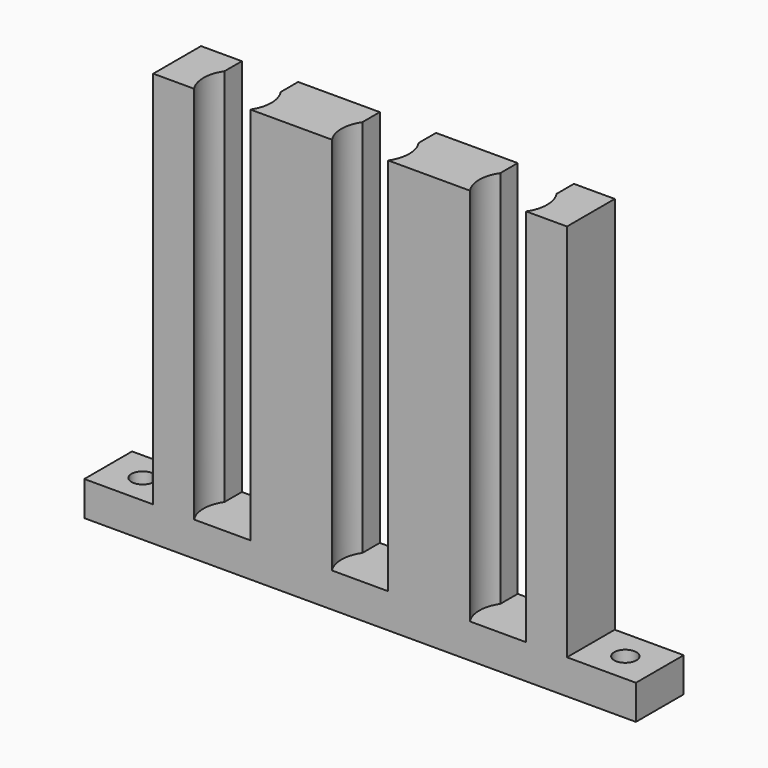
from build123d import *

# Parameters (mm, degrees)
F0_W         = 76.2
F0_H         = 11
F1_DEPTH     = 76.2
F2_R         = 6.25
F3_DEPTH     = 69.85
F4_TEXT_SIZE = 5.2916666667
F5_DEPTH     = 0.5
F6_W         = 11
F6_H         = 6.35
F7_DEPTH     = 12.7
F8_W         = 11
F8_H         = 6.35
F9_DEPTH     = 12.7
F10_R        = 2.05
F11_DEPTH    = 6.35
F12_W        = 10.3561575886
F12_H        = 4
F13_DEPTH    = 69.85


# Not quite as in the source:
# - Text() gives the source's letters only with a copy of the font that has no kerning and outlines rounded to 1/6400 em; it was checked with that copy


with BuildPart() as f1:
    # F0 (on Top) → F1 (new body)
    with BuildSketch(Plane.XY):
        Rectangle(F0_W, F0_H)
    extrude(amount=F1_DEPTH)

    # F2 (on face) → F3 (cut)
    with BuildSketch(Plane.XY.offset(76.2)):
        with BuildLine():
            ThreePointArc((0, 4.25), (-4.4194173824, -6.4194173824), (6.25, -2))
            ThreePointArc((6.25, -2), (4.4194173824, 2.4194173824), (0, 4.25))
        make_face()
        with Locations((-25.4, -2)):
            Circle(F2_R)
        with Locations((25.4, -2)):
            Circle(F2_R)
    extrude(amount=-F3_DEPTH, mode=Mode.SUBTRACT)

    # F4 (on face) → F5 (cut)
    with BuildSketch(Plane(origin=(0, 5.5, 0), x_dir=(-1, 0, 0), z_dir=(0, 1, 0))):
        with Locations((-26.8469244572, 1.5566079867)):
            Text('1', F4_TEXT_SIZE, font='Open Sans', text_align=(TextAlign.LEFT, TextAlign.BOTTOM))
        with Locations((-1.5416732874, 1.5566079867)):
            Text('2', F4_TEXT_SIZE, font='Open Sans', text_align=(TextAlign.LEFT, TextAlign.BOTTOM))
        with Locations((24.0893187388, 1.5566079867)):
            Text('3', F4_TEXT_SIZE, font='Open Sans', text_align=(TextAlign.LEFT, TextAlign.BOTTOM))
    extrude(amount=-F5_DEPTH, mode=Mode.SUBTRACT)

    # F6 (on face) → F7 (join)
    with BuildSketch(Plane.YZ.offset(38.1)):
        with Locations((0, 3.175)):
            Rectangle(F6_W, F6_H)
    extrude(amount=F7_DEPTH)

    # F8 (on face) → F9 (join)
    with BuildSketch(Plane(origin=(-38.1, 0, 0), x_dir=(0, -1, 0), z_dir=(-1, 0, 0))):
        with Locations((0, 3.175)):
            Rectangle(F8_W, F8_H)
    extrude(amount=F9_DEPTH)

    # F10 (on face) → F11 (cut, through all)
    with BuildSketch(Plane.XY.offset(6.35)):
        with BuildLine():
            ThreePointArc((-44.45, -2.05), (-43.0004310986, -1.4495689014), (-42.4, 0))
            ThreePointArc((-42.4, 0), (-43.0004310986, 1.4495689014), (-44.45, 2.05))
            Line((-44.45, 2.05), (-44.45, -2.05))
        make_face()
        with BuildLine():
            Line((-44.45, -2.05), (-44.45, 2.05))
            ThreePointArc((-44.45, 2.05), (-46.5, 0), (-44.45, -2.05))
        make_face()
        with Locations((44.45, 0)):
            Circle(F10_R)
    extrude(amount=-F11_DEPTH, mode=Mode.SUBTRACT)

    # F12 (on face) → F13 (cut, through all)
    with BuildSketch(Plane.XY.offset(76.2)):
        with Locations((-25.4, 3.5)):
            Rectangle(F12_W, F12_H)
        with Locations((0, 3.5)):
            Rectangle(F12_W, F12_H)
        with Locations((25.4, 3.5)):
            Rectangle(F12_W, F12_H)
    extrude(amount=-F13_DEPTH, mode=Mode.SUBTRACT)


solid = f1.part
